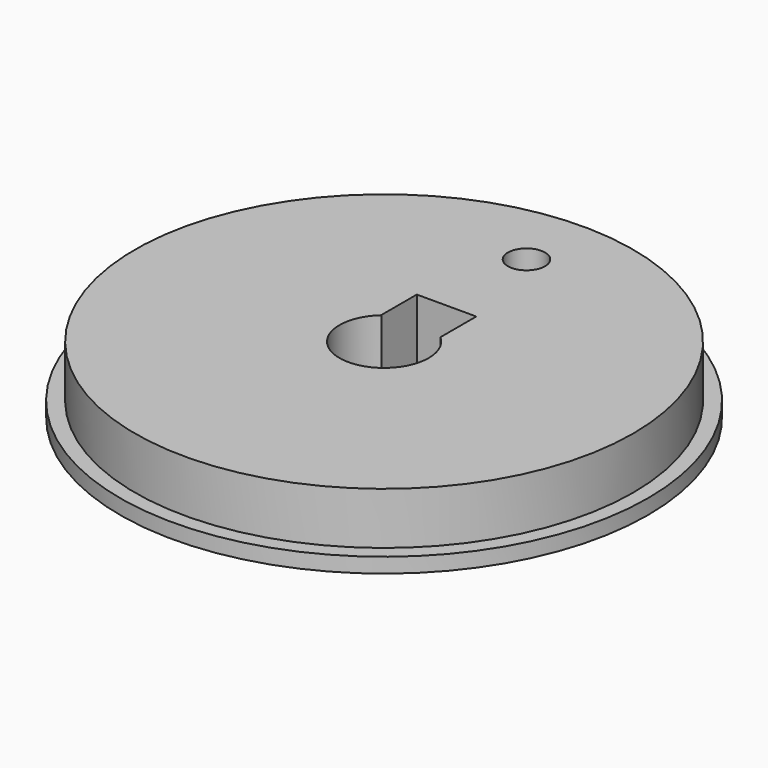
from build123d import *

# Parameters (mm, degrees)
F0_R     = 16.75
F0_R_2   = 1.25
F1_DEPTH = 4.5
F0_R_3   = 17.75
F2_DEPTH = 1


# Not quite as in the source:
# - a feature names something its author has since deleted; it is built from what else it names


with BuildPart() as f1:
    # F0 (on Top) → F1 (new body)
    with BuildSketch(Plane.XY):
        Circle(F0_R)
        with BuildLine():
            ThreePointArc((1.9843134833, 2.25), (2.7343134833, 1.2343134833), (3, 0))
            ThreePointArc((3, 0), (-1.2343134833, -2.7343134833), (-1.9843134833, 2.25))
            Line((-1.9843134833, 2.25), (-2, 2.25))
            Line((-2, 2.25), (-2, 5.25))
            Line((-2, 5.25), (2, 5.25))
            Line((2, 5.25), (2, 2.25))
            Line((2, 2.25), (1.9843134833, 2.25))
        make_face(mode=Mode.SUBTRACT)
        with Locations((0, 11.9703095406)):
            Circle(F0_R_2, mode=Mode.SUBTRACT)
    extrude(amount=F1_DEPTH)

    # F0 (on Top) → F2 (join)
    with BuildSketch(Plane.XY):
        Circle(F0_R_3)
        Circle(F0_R, mode=Mode.SUBTRACT)
    extrude(amount=F2_DEPTH)


solid = f1.part
